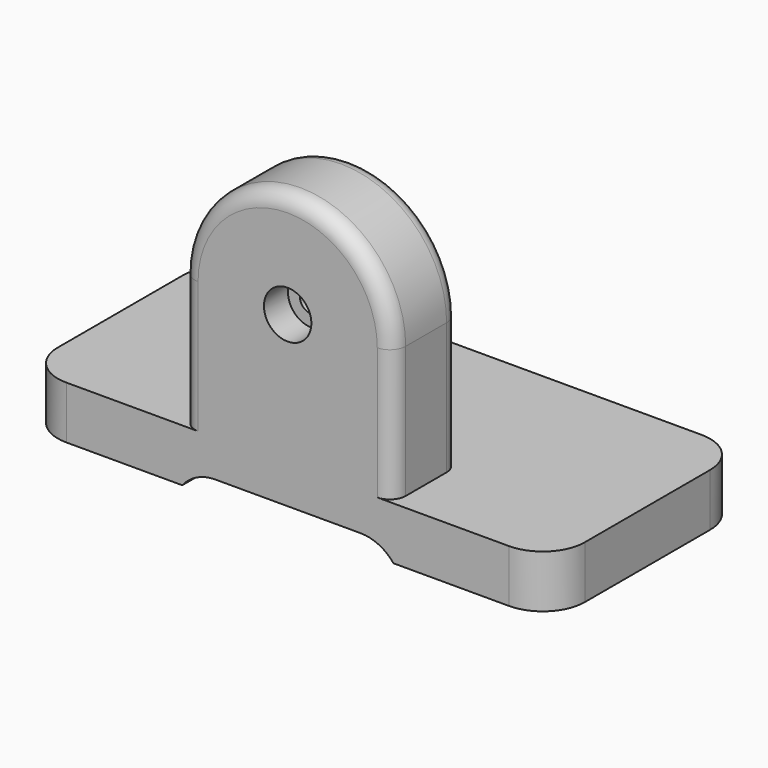
from build123d import *

# Parameters (mm, degrees)
F0_W          = 100
F0_H          = 40
F1_DEPTH      = 10
F3_DEPTH      = 10
F4_W          = 40.0635205954
F4_H          = 3
F5_DEPTH      = 40.001
F6_R          = 2.25
F7_DEPTH      = 10.001
F8_R          = 4.5
F10_DEPTH     = 5.7
F11_T1_DEPTH  = 45.7
F11_T3_DEPTH  = 45.7
F11_T5_DEPTH  = 50
F11_T7_DEPTH  = 50
F11_T9_DEPTH  = 50
F11_T11_DEPTH = 50
F12_R         = 3


# Not quite as in the source:
# - a fillet or chamfer that OpenCascade refuses, or shapes differently, is made with other operations: its cross-section is extruded or revolved along the edge and cut away or added
# - the program builds the solid bodies; features that only make, move or delete a surface that nothing else refers to are left out


with BuildPart() as f1:
    # F0 (on Top) → F1 (new body)
    with BuildSketch(Plane.XY):
        with Locations((-50, 20)):
            Rectangle(F0_W, F0_H)
    extrude(amount=F1_DEPTH)

    # F2 (on face) → F3 (join)
    with BuildSketch(Plane.XZ):
        with BuildLine():
            ThreePointArc((-30, 35), (-50, 55), (-70, 35))
            Line((-70, 35), (-70, 0))
            Line((-70, 0), (-30, 0))
            Line((-30, 0), (-30, 35))
        make_face()
    extrude(amount=-F3_DEPTH)

    # F4 (on face) → F5 (cut, through all)
    with BuildSketch(Plane.XZ):
        with Locations((-49.9682397023, 1.5)):
            Rectangle(F4_W, F4_H)
    extrude(amount=-F5_DEPTH, mode=Mode.SUBTRACT)

    # F6 (on face) → F7 (cut, through all)
    with BuildSketch(Plane(origin=(0, 10, 0), x_dir=(-1, 0, 0), z_dir=(0, 1, 0))):
        with Locations((50, 35)):
            Circle(F6_R)
    extrude(amount=-F7_DEPTH, mode=Mode.SUBTRACT)

    # F8 (on face) → F10 (join)
    with BuildSketch(Plane.XZ):
        with BuildLine():
            Line((-100, 10), (-100, 0))
            Line((-100, 0), (-70, 0))
            Line((-70, 0), (-70, 3))
            Line((-70, 3), (-29.9364794046, 3))
            Line((-29.9364794046, 3), (-29.9364794046, 0))
            Line((-29.9364794046, 0), (0, 0))
            Line((0, 0), (0, 10))
            Line((0, 10), (-30, 10))
            Line((-30, 10), (-30, 35))
            ThreePointArc((-30, 35), (-50, 55), (-70, 35))
            Line((-70, 35), (-70, 10))
            Line((-70, 10), (-100, 10))
        make_face()
        with Locations((-50, 35)):
            Circle(F8_R, mode=Mode.SUBTRACT)
    extrude(amount=F10_DEPTH)

    # F11: fillet of radius 8 on 8 edges, made by hand

    # F11_s2 → F11_t1 (join)
    with BuildSketch(Plane.XZ.offset(-40)):
        with BuildLine():
            ThreePointArc((-29.9364794046, 0), (-32.7173757878, 2.2111025509), (-36.181477403, 3))
            Line((-36.181477403, 3), (-29.9364794046, 3))
            Line((-29.9364794046, 3), (-29.9364794046, 0))
        make_face()
    extrude(amount=F11_T1_DEPTH)

    # F11_s4 → F11_t3 (join)
    with BuildSketch(Plane.XZ.offset(-40)):
        with BuildLine():
            ThreePointArc((-70, 0), (-67.2191036167, 2.2111025509), (-63.7550020016, 3))
            Line((-63.7550020016, 3), (-70, 3))
            Line((-70, 3), (-70, 0))
        make_face()
    extrude(amount=F11_T3_DEPTH)

    # F11_s6 → F11_t5 (cut)
    with BuildSketch(Plane.XY.offset(-20)):
        with BuildLine():
            ThreePointArc((-92, -5.7), (-97.6568542495, -3.3568542495), (-100, 2.3))
            Line((-100, 2.3), (-100, -5.7))
            Line((-100, -5.7), (-92, -5.7))
        make_face()
    extrude(amount=F11_T5_DEPTH, mode=Mode.SUBTRACT)

    # F11_s8 → F11_t7 (cut)
    with BuildSketch(Plane.XY.offset(-20)):
        with BuildLine():
            ThreePointArc((-8, -5.7), (-2.3431457505, -3.3568542495), (0, 2.3))
            Line((0, 2.3), (0, -5.7))
            Line((0, -5.7), (-8, -5.7))
        make_face()
    extrude(amount=F11_T7_DEPTH, mode=Mode.SUBTRACT)

    # F11_s10 → F11_t9 (cut)
    with BuildSketch(Plane.XY.offset(-20)):
        with BuildLine():
            ThreePointArc((-8, 40), (-2.3431457505, 37.6568542495), (0, 32))
            Line((0, 32), (0, 40))
            Line((0, 40), (-8, 40))
        make_face()
    extrude(amount=F11_T9_DEPTH, mode=Mode.SUBTRACT)

    # F11_s12 → F11_t11 (cut)
    with BuildSketch(Plane.XY.offset(-20)):
        with BuildLine():
            ThreePointArc((-92, 40), (-97.6568542495, 37.6568542495), (-100, 32))
            Line((-100, 32), (-100, 40))
            Line((-100, 40), (-92, 40))
        make_face()
    extrude(amount=F11_T11_DEPTH, mode=Mode.SUBTRACT)

    # F12
    f12_edges = [f1.edges().sort_by_distance(p)[0] for p in [
        (-30, -5.7, 22.5),
        (-50, -5.7, 55),
        (-50, 10, 55),
        (-70, -5.7, 22.5),
        (-30, 10, 22.5),
        (-70, 10, 22.5),
    ]]
    fillet(f12_edges, radius=F12_R)


solid = f1.part
